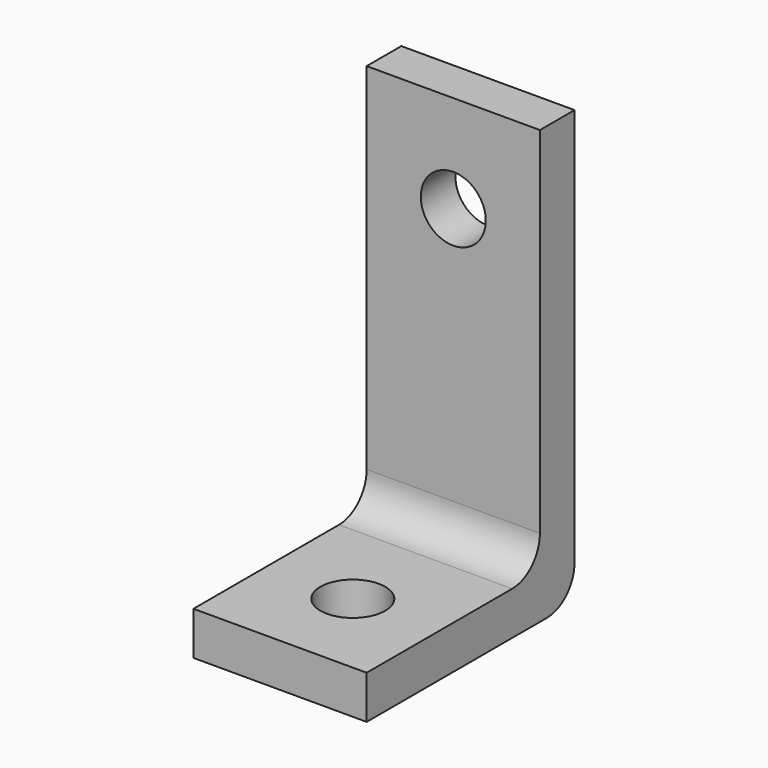
from build123d import *

# Parameters (mm, degrees)
F0_W     = 12.7
F0_H     = 6.35
F1_DEPTH = 38.1
F0_H_2   = 57.15
F2_DEPTH = 6.35
F3_R     = 5.08
F5_D     = 9.525
F6_D     = 9.525


# Not quite as in the source:
# - a length typed as a fraction of an inch, garbled in the dataset ("3 / 203.2 mm" for 3/8 in), is restored


with BuildPart() as f1:
    # F0 (on Front) → F1 (new body)
    with BuildSketch(Plane.XZ):
        with Locations((6.35, 3.175)):
            Rectangle(F0_W, F0_H)
        with Locations((19.05, 3.175)):
            Rectangle(F0_W, F0_H)
    extrude(amount=F1_DEPTH)

    # F0 (on Front) → F2 (join)
    with BuildSketch(Plane.XZ):
        with Locations((6.35, 3.175)):
            Rectangle(F0_W, F0_H)
        with Locations((19.05, 3.175)):
            Rectangle(F0_W, F0_H)
        with Locations((6.35, 34.925)):
            Rectangle(F0_W, F0_H_2)
        with Locations((19.05, 34.925)):
            Rectangle(F0_W, F0_H_2)
    extrude(amount=F2_DEPTH)

    # F3
    f3_edges = [f1.edges().sort_by_distance(p)[0] for p in [
        (12.7, -6.35, 6.35),
        (12.7, 0, 0),
    ]]
    fillet(f3_edges, radius=F3_R)

    # F5 (through all)
    with Locations(Plane.XY.offset(6.35)):
        with Locations((12.7, -24.765)):
            Hole(F5_D / 2)

    # F6 (through all)
    with Locations(Plane(origin=(0, 0, 0), x_dir=(1, 0, 0), z_dir=(0, 1, 0))):
        with Locations((12.7, -49.2125)):
            Hole(F6_D / 2)


solid = f1.part
